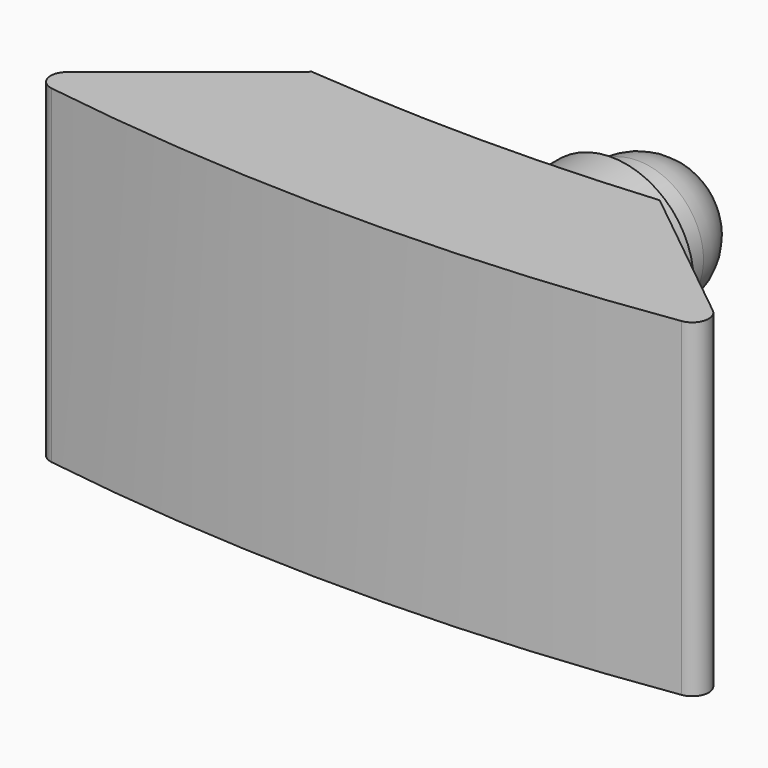
from build123d import *

# Parameters (mm, degrees)
F0_R          = 5
F1_DEPTH      = 10
F2_R          = 4
F3_DEPTH      = 6
F4_R          = 4
F6_DEPTH      = 10
F6_DEPTH_BACK = 10
F7_T4_DEPTH   = 20
F7_S5_R       = 120
F7_T6_DEPTH   = 12
F7_T10_DEPTH  = 20
F7_S11_R      = 120
F7_T12_DEPTH  = 12
F9_DEPTH      = 25
F10_R         = 1


# Not quite as in the source:
# - a fillet or chamfer that OpenCascade refuses, or shapes differently, is made with other operations: its cross-section is extruded or revolved along the edge and cut away or added


with BuildPart() as f1:
    # F0 (on Front) → F1 (new body)
    with BuildSketch(Plane.XZ):
        Circle(F0_R)
    extrude(amount=F1_DEPTH)

    # F2 (on face) → F3 (join)
    with BuildSketch(Plane(origin=(0, 0, 0), x_dir=(-1, 0, 0), z_dir=(0, 1, 0))):
        Circle(F2_R)
    extrude(amount=F3_DEPTH)

    # F4
    f4_edges = [f1.edges().sort_by_distance(p)[0] for p in [
        (4, 6, 0),
    ]]
    fillet(f4_edges, radius=F4_R)

    # F5 (on Top) → F6 (join, two sides)
    with BuildSketch(Plane.XY) as f6_sk:
        with BuildLine():
            ThreePointArc((10.4586891297, -9.543363771), (0, -10), (-10.4586891297, -9.543363771))
            Line((-10.4586891297, -9.543363771), (-10.8944678435, -14.5243372615))
            ThreePointArc((-10.8944678435, -14.5243372615), (-16.3157740275, -13.9306076717), (-21.7060222084, -13.1009691265))
            Line((-21.7060222084, -13.1009691265), (-22.5742630967, -18.0250078916))
            ThreePointArc((-22.5742630967, -18.0250078916), (0, -20), (22.5742630967, -18.0250078916))
            Line((22.5742630967, -18.0250078916), (21.7060222084, -13.1009691265))
            ThreePointArc((21.7060222084, -13.1009691265), (16.3157740275, -13.9306076717), (10.8944678435, -14.5243372615))
            Line((10.8944678435, -14.5243372615), (10.4586891297, -9.543363771))
        make_face()
    extrude(amount=F6_DEPTH)
    extrude(f6_sk.sketch, amount=-F6_DEPTH_BACK)

    # F7: chamfer of 5 on 2 edges, made by hand


with BuildPart() as f7_tool2:
    # F7_s3 → F7_t4 (new body)
    with BuildSketch(Plane.XY.offset(-10)):
        with BuildLine():
            Line((-16.0735207845, -13.962260102), (-10.4496064627, -9.4395484116))
            Line((-10.4496064627, -9.4395484116), (-10.8944678435, -14.5243372615))
            ThreePointArc((-10.8944678435, -14.5243372615), (-13.5571939783, -14.262635138), (-16.0735207845, -13.962260102))
        make_face()
    extrude(amount=F7_T4_DEPTH)

    # F7_s5 → F7_t6 (cut, symmetric)
    with BuildSketch(Plane.XY):
        with Locations((0, 110)):
            Circle(F7_S5_R)
    extrude(amount=F7_T6_DEPTH, both=True, mode=Mode.SUBTRACT)


with BuildPart() as f1_1:
    add(f1.part)

    # F7_t1: union F7_tool2
    add(f7_tool2.part)


with BuildPart() as f7_tool8:
    # F7_s9 → F7_t10 (new body)
    with BuildSketch(Plane.XY.offset(10)):
        with BuildLine():
            Line((10.4496064627, -9.4395484116), (16.0735207845, -13.962260102))
            ThreePointArc((16.0735207845, -13.962260102), (13.5571939783, -14.262635138), (10.8944678435, -14.5243372615))
            Line((10.8944678435, -14.5243372615), (10.4496064627, -9.4395484116))
        make_face()
    extrude(amount=-F7_T10_DEPTH)

    # F7_s11 → F7_t12 (cut, symmetric)
    with BuildSketch(Plane.XY):
        with Locations((0, 110)):
            Circle(F7_S11_R)
    extrude(amount=F7_T12_DEPTH, both=True, mode=Mode.SUBTRACT)


with BuildPart() as f1_2:
    add(f1_1.part)

    # F7_t7: union F7_tool8
    add(f7_tool8.part)

    # F8 (on face) → F9 (cut)
    with BuildSketch(Plane.XY.offset(10)):
        Polygon((-22.1401426525, -18.8409940359), (-16.0735207845, -13.962260102), (-26.2115597725, -8.7402015924), (-26.2115597725, -18.8409940359), align=None)
        Polygon((26.2115597725, -8.7402015924), (16.0735207845, -13.962260102), (22.1401426525, -18.8409940359), (26.2115597725, -18.8409940359), align=None)
    extrude(amount=-F9_DEPTH, mode=Mode.SUBTRACT)

    # F10
    f10_edges = [f1_2.edges().sort_by_distance(p)[0] for p in [
        (-21.380167, -18.229827, 0),
        (21.380167, -18.229827, 0),
    ]]
    fillet(f10_edges, radius=F10_R)


solid = f1_2.part
